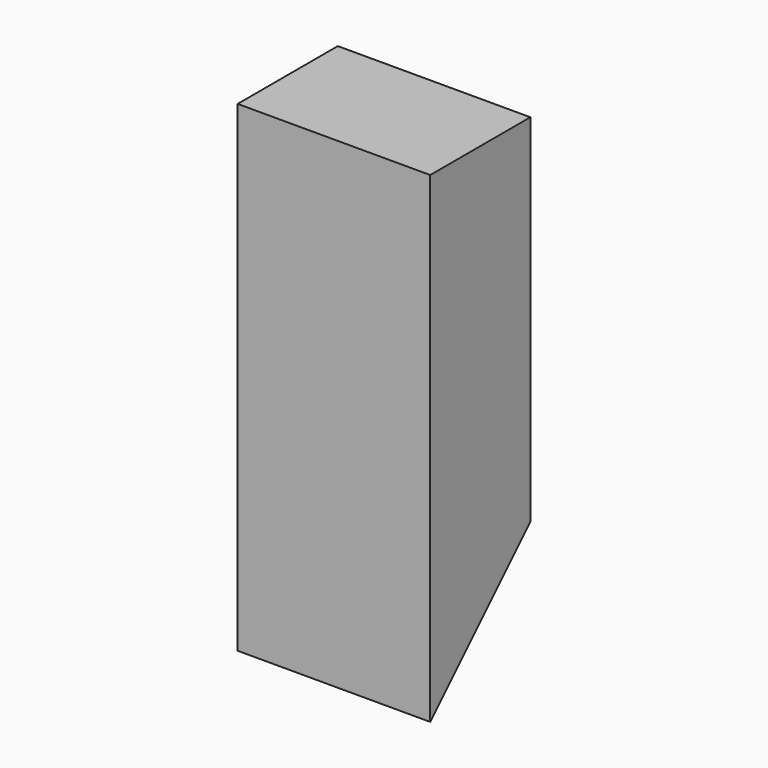
from build123d import *

# Parameters (mm, degrees)
F0_W     = 50.8
F0_H     = 127
F1_DEPTH = 33.02
F2_SIZE  = 33.01999


# Not quite as in the source:
# - a fillet or chamfer is up to 0.001 mm smaller than in the source, because OpenCascade refuses the exact size


with BuildPart() as f1:
    # F0 (on Front) → F1 (new body)
    with BuildSketch(Plane.XZ):
        Rectangle(F0_W, F0_H)
    extrude(amount=F1_DEPTH)

    # F2 (size 33.02 in the source; OpenCascade refuses exactly that, so slightly less here)
    f2_edges = [f1.edges().sort_by_distance(p)[0] for p in [
        (0, 0, -63.5),
    ]]
    chamfer(f2_edges, length=F2_SIZE)


solid = f1.part
